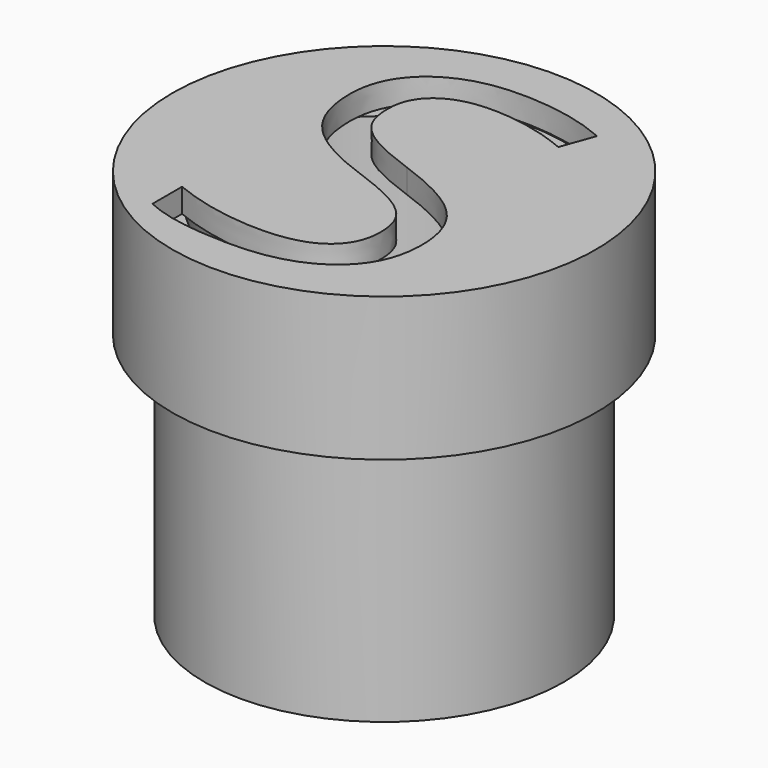
from build123d import *

# Parameters (mm, degrees)
F4_TEXT_SIZE = 38.6589048811
F5_DEPTH     = 2


# Not quite as in the source:
# - Text() gives the source's letters only with a copy of the font that has no kerning and outlines rounded to 1/6400 em; it was checked with that copy


with BuildPart() as f1:
    # F0 (on Front) → F1 (revolve)
    with BuildSketch(Plane.XZ):
        Polygon((-15, 0), (0, 0), (0, 2), (-13, 2), (-13, 30), (-15, 30), (-15, 21.6), (-14.2, 20.8), (-15, 20), align=None)
    revolve(axis=Axis((0, 0, 22.6602833718), (0, 0, 1)))


with BuildPart() as f3:
    # F2 (on Front) → F3 (revolve)
    with BuildSketch(Plane.XZ):
        Polygon((-15.7, 30.7), (0, 30.7), (0, 32.7), (-17.7, 32.7), (-17.7, 20.7), (-15.7, 20.7), (-14.9, 20.7), (-15.7, 21.5), align=None)
    revolve(axis=Axis((0, 0, 54.083638823), (0, 0, 1)))

    # F4 (on face) → F5 (cut, through all)
    with BuildSketch(Plane.XY.offset(32.7)):
        with Locations((-10.9362417636, -13.9172057572)):
            Text('S', F4_TEXT_SIZE, font='Open Sans', text_align=(TextAlign.LEFT, TextAlign.BOTTOM))
    extrude(amount=-F5_DEPTH, mode=Mode.SUBTRACT)


solid = Compound([f1.part, f3.part])
